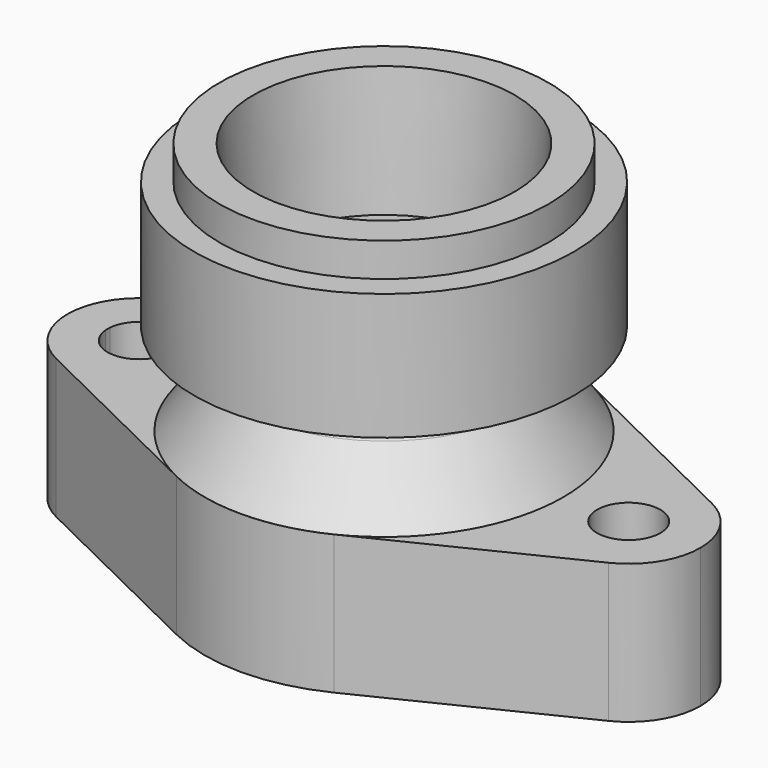
from build123d import *

# Parameters (mm, degrees)
F1_DEPTH  = 33
F3_R      = 40
F4_DEPTH  = 3
F6_R      = 45
F6_R_2    = 34.1243185103
F7_DEPTH  = 38
F8_R      = 45
F8_R_2    = 39
F9_DEPTH  = 8
F10_R     = 31
F11_DEPTH = 30
F11_TAPER = 3.85
F12_R     = 26
F13_DEPTH = 42


with BuildPart() as f1:
    # F0 (on Top) → F1 (new body)
    with BuildSketch(Plane.XY):
        with BuildLine():
            ThreePointArc((-42.0797413793, -5.9619934125), (-42.5, 0), (-42.0797413793, 5.9619934125))
            ThreePointArc((-42.0797413793, 5.9619934125), (-51.7160080676, 15.7959312924), (-65.474137931, 15.2688330329))
            Line((-65.474137931, 15.2688330329), (-65.474137931, 0.6223039353))
            ThreePointArc((-65.474137931, 0.6223039353), (-57.6885794505, 7.4935316935), (-50.5, 0))
            ThreePointArc((-50.5, 0), (-57.6885794505, -7.4935316935), (-65.474137931, -0.6223039353))
            Line((-65.474137931, -0.6223039353), (-65.474137931, -15.2688330329))
            ThreePointArc((-65.474137931, -15.2688330329), (-51.7160080676, -15.7959312924), (-42.0797413793, -5.9619934125))
        make_face()
        with BuildLine():
            ThreePointArc((-18.6853448276, -38.1720825824), (-34.3870816807, -24.9755603237), (-42.0797413793, -5.9619934125))
            ThreePointArc((-42.0797413793, -5.9619934125), (-51.7160080676, -15.7959312924), (-65.474137931, -15.2688330329))
            Line((-65.474137931, -15.2688330329), (-18.6853448276, -38.1720825824))
        make_face()
        with BuildLine():
            Line((-65.474137931, 0.6223039353), (-65.474137931, 15.2688330329))
            ThreePointArc((-65.474137931, 15.2688330329), (-75, 0), (-65.474137931, -15.2688330329))
            Line((-65.474137931, -15.2688330329), (-65.474137931, -0.6223039353))
            ThreePointArc((-65.474137931, -0.6223039353), (-65.5, 0), (-65.474137931, 0.6223039353))
        make_face()
        with BuildLine():
            Line((65.474137931, 15.2688330329), (18.6853448276, 38.1720825824))
            ThreePointArc((18.6853448276, 38.1720825824), (34.3870816807, 24.9755603237), (42.0797413793, 5.9619934125))
            ThreePointArc((42.0797413793, 5.9619934125), (51.7160080676, 15.7959312924), (65.474137931, 15.2688330329))
        make_face()
        with BuildLine():
            ThreePointArc((75, 0), (72.4232511042, 8.9983235987), (65.474137931, 15.2688330329))
            Line((65.474137931, 15.2688330329), (65.474137931, 0.6223039353))
            ThreePointArc((65.474137931, 0.6223039353), (65.4935316935, 0.3114205495), (65.5, 0))
            ThreePointArc((65.5, 0), (65.4935316935, -0.3114205495), (65.474137931, -0.6223039353))
            Line((65.474137931, -0.6223039353), (65.474137931, -15.2688330329))
            ThreePointArc((65.474137931, -15.2688330329), (72.4232511042, -8.9983235987), (75, 0))
        make_face()
        with BuildLine():
            ThreePointArc((42.0797413793, 5.9619934125), (34.3870816807, 24.9755603237), (18.6853448276, 38.1720825824))
            ThreePointArc((18.6853448276, 38.1720825824), (0, 42.5), (-18.6853448276, 38.1720825824))
            ThreePointArc((-18.6853448276, 38.1720825824), (-34.3870816807, 24.9755603237), (-42.0797413793, 5.9619934125))
            ThreePointArc((-42.0797413793, 5.9619934125), (-41.2721131557, 3.0294886902), (-41, 0))
            ThreePointArc((-41, 0), (-41.2721131557, -3.0294886902), (-42.0797413793, -5.9619934125))
            ThreePointArc((-42.0797413793, -5.9619934125), (-34.3870816807, -24.9755603237), (-18.6853448276, -38.1720825824))
            ThreePointArc((-18.6853448276, -38.1720825824), (0, -42.5), (18.6853448276, -38.1720825824))
            ThreePointArc((18.6853448276, -38.1720825824), (34.3870816807, -24.9755603237), (42.0797413793, -5.9619934125))
            ThreePointArc((42.0797413793, -5.9619934125), (41, 0), (42.0797413793, 5.9619934125))
        make_face()
        with BuildLine():
            ThreePointArc((42.5, 0), (42.3948051571, 2.9883934965), (42.0797413793, 5.9619934125))
            ThreePointArc((42.0797413793, 5.9619934125), (41, 0), (42.0797413793, -5.9619934125))
            ThreePointArc((42.0797413793, -5.9619934125), (42.3948051571, -2.9883934965), (42.5, 0))
        make_face()
        with BuildLine():
            ThreePointArc((65.474137931, 15.2688330329), (51.7160080676, 15.7959312924), (42.0797413793, 5.9619934125))
            ThreePointArc((42.0797413793, 5.9619934125), (42.3948051571, 2.9883934965), (42.5, 0))
            ThreePointArc((42.5, 0), (42.3948051571, -2.9883934965), (42.0797413793, -5.9619934125))
            ThreePointArc((42.0797413793, -5.9619934125), (51.7160080676, -15.7959312924), (65.474137931, -15.2688330329))
            Line((65.474137931, -15.2688330329), (65.474137931, -0.6223039353))
            ThreePointArc((65.474137931, -0.6223039353), (50.5, 0), (65.474137931, 0.6223039353))
            Line((65.474137931, 0.6223039353), (65.474137931, 15.2688330329))
        make_face()
        with BuildLine():
            ThreePointArc((65.474137931, -15.2688330329), (51.7160080676, -15.7959312924), (42.0797413793, -5.9619934125))
            ThreePointArc((42.0797413793, -5.9619934125), (34.3870816807, -24.9755603237), (18.6853448276, -38.1720825824))
            Line((18.6853448276, -38.1720825824), (65.474137931, -15.2688330329))
        make_face()
        with BuildLine():
            ThreePointArc((-42.0797413793, 5.9619934125), (-34.3870816807, 24.9755603237), (-18.6853448276, 38.1720825824))
            Line((-18.6853448276, 38.1720825824), (-65.474137931, 15.2688330329))
            ThreePointArc((-65.474137931, 15.2688330329), (-51.7160080676, 15.7959312924), (-42.0797413793, 5.9619934125))
        make_face()
        with BuildLine():
            ThreePointArc((-41, 0), (-41.2721131557, 3.0294886902), (-42.0797413793, 5.9619934125))
            ThreePointArc((-42.0797413793, 5.9619934125), (-42.5, 0), (-42.0797413793, -5.9619934125))
            ThreePointArc((-42.0797413793, -5.9619934125), (-41.2721131557, -3.0294886902), (-41, 0))
        make_face()
    extrude(amount=F1_DEPTH)

    # F3 (on face) → F4 (cut)
    with BuildSketch(Plane.XY):
        Circle(F3_R)
    extrude(amount=F4_DEPTH, mode=Mode.SUBTRACT)

    # F2 (on Front) → F5 (revolve)
    with BuildSketch(Plane.XZ):
        with BuildLine():
            Line((-42.499996424, 32.9825655057), (0, 33))
            Line((0, 33), (0, 55))
            Line((0, 55), (-27.083222819, 55))
            Line((-27.083222819, 55), (-34.1243185103, 55))
            ThreePointArc((-34.1243185103, 55), (-31.4867427552, 51.7572794356), (-32.2335459741, 47.6445762521))
            Line((-32.2335459741, 47.6445762521), (-42.499996424, 32.9825655057))
        make_face()
    revolve(axis=Axis((0, 0, 44), (0, 0, 1)))

    # F6 (on face) → F7 (join)
    with BuildSketch(Plane.XY.offset(55)):
        Circle(F6_R)
        Circle(F6_R_2, mode=Mode.SUBTRACT)
        Circle(F6_R_2)
    extrude(amount=F7_DEPTH)

    # F8 (on face) → F9 (cut)
    with BuildSketch(Plane.XY.offset(93)):
        Circle(F8_R)
        Circle(F8_R_2, mode=Mode.SUBTRACT)
    extrude(amount=-F9_DEPTH, mode=Mode.SUBTRACT)

    # F10 (on face) → F11 (cut)
    with BuildSketch(Plane.XY.offset(93)):
        Circle(F10_R)
    extrude(amount=-F11_DEPTH, taper=F11_TAPER, mode=Mode.SUBTRACT)

    # F12 (on face) → F13 (cut)
    with BuildSketch(Plane.XY.offset(63)):
        Circle(F12_R)
    extrude(amount=-F13_DEPTH, mode=Mode.SUBTRACT)


solid = f1.part
